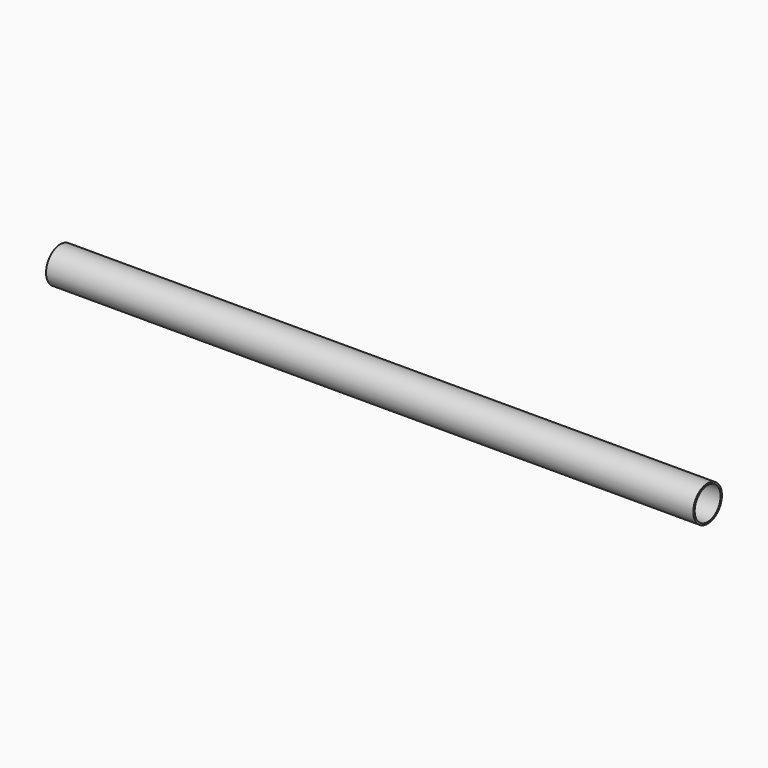
from build123d import *

# Parameters (mm, degrees)
F1_R     = 84.1375
F1_R_2   = 76.2
F2_DEPTH = 3048


# Not quite as in the source:
# - a variable given as a bare number and used for a length is read in inches; the dataset says mm whatever the document's units were


with BuildPart() as f2:
    # F1 (on Right) → F2 (new body)
    with BuildSketch(Plane.YZ):
        Circle(F1_R)
        Circle(F1_R_2, mode=Mode.SUBTRACT)
    extrude(amount=-F2_DEPTH)


solid = f2.part
